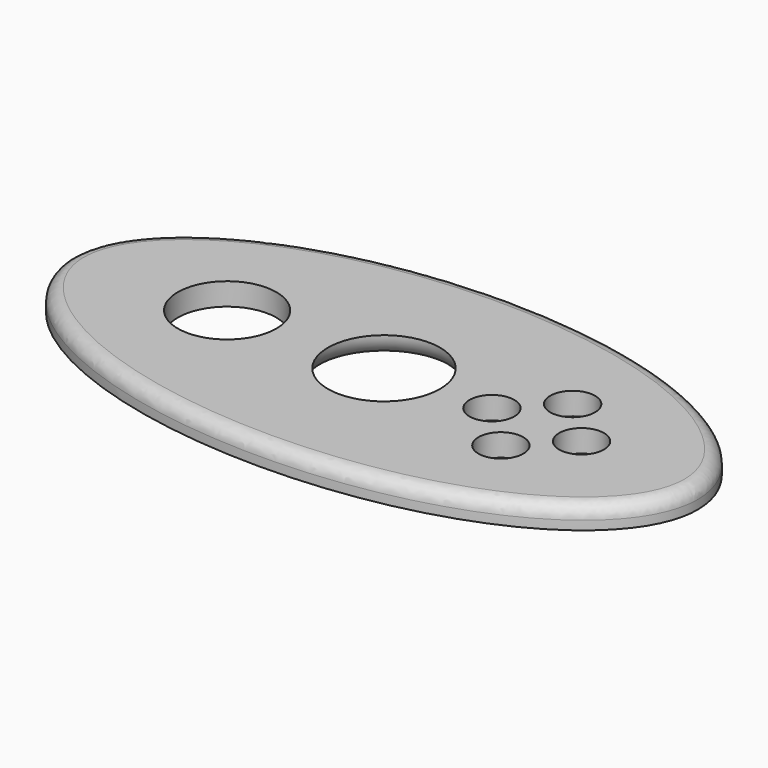
from build123d import *

# Parameters (mm, degrees)
F0_R     = 5
F0_R_2   = 11
F0_R_3   = 12.5
F1_DEPTH = 5
F2_R     = 4.99999
F3_R     = 3


# Not quite as in the source:
# - a fillet or chamfer is up to 0.001 mm smaller than in the source, because OpenCascade refuses the exact size


with BuildPart() as f1:
    # F0 (on Top) → F1 (new body)
    with BuildSketch(Plane.XY):
        with BuildLine():
            add(Edge.make_bspline(
                [(70, 0), (70, 60.6217782649), (-35, 30.3108891325), (-140, 0), (-35, -30.3108891325), (70, -60.6217782649), (70, 0)],
                knots=[0, 0, 0, 2.0943951024, 2.0943951024, 4.1887902048, 4.1887902048, 6.2831853072, 6.2831853072, 6.2831853072], degree=2, weights=[1, 0.5, 1, 0.5, 1, 0.5, 1]))
        make_face()
        with Locations((34.0825345158, -10)):
            Circle(F0_R, mode=Mode.SUBTRACT)
        with Locations((-35, 0)):
            Circle(F0_R_2, mode=Mode.SUBTRACT)
        Circle(F0_R_3, mode=Mode.SUBTRACT)
        with Locations((24.0825345158, 0)):
            Circle(F0_R, mode=Mode.SUBTRACT)
        with Locations((34.0825345158, 10)):
            Circle(F0_R, mode=Mode.SUBTRACT)
        with Locations((44.0825345158, 0)):
            Circle(F0_R, mode=Mode.SUBTRACT)
    extrude(amount=F1_DEPTH)

    # F2 (radius 5 in the source; OpenCascade refuses exactly that, so slightly less here)
    f2_edges = [f1.edges().sort_by_distance(p)[0] for p in [
        (-12.5, 0, 0),
    ]]
    fillet(f2_edges, radius=F2_R)

    # F3
    f3_edges = [f1.edges().sort_by_distance(p)[0] for p in [
        (-70, 9e-06, 5),
    ]]
    fillet(f3_edges, radius=F3_R)


solid = f1.part
